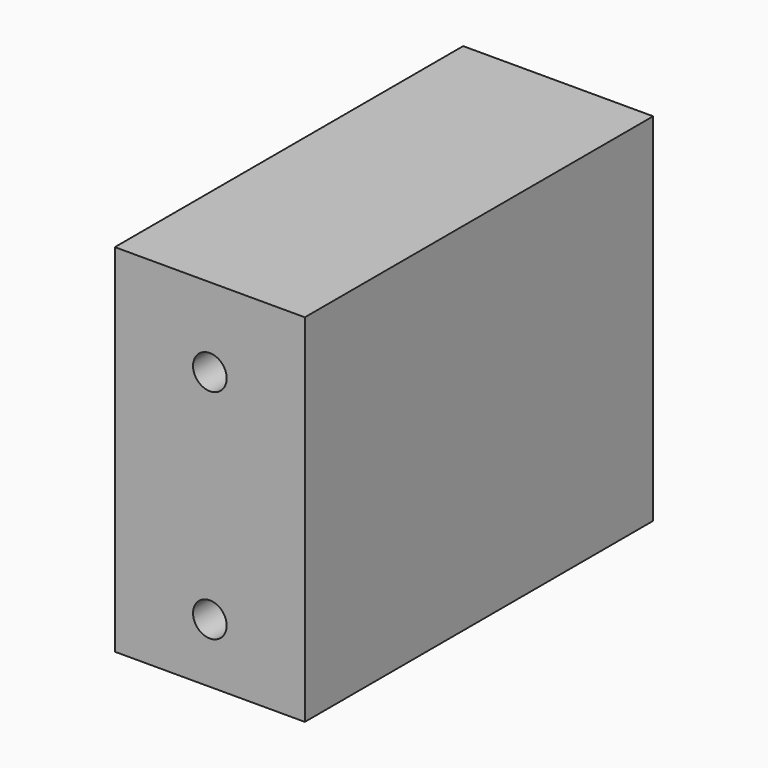
from build123d import *

# Parameters (mm, degrees)
F0_W     = 48
F0_H     = 90
F1_DEPTH = 110
F3_D     = 8.5


# Not quite as in the source:
# - the program builds the solid bodies; features that only make, move or delete a surface that nothing else refers to are left out


with BuildPart() as f1:
    # F0 (on Front) → F1 (new body)
    with BuildSketch(Plane.XZ):
        with Locations((24, 45)):
            Rectangle(F0_W, F0_H)
    extrude(amount=F1_DEPTH)

    # F3 (through all)
    with Locations(Plane.XZ.offset(110)):
        with Locations((24, 70), (24, 15)):
            Hole(F3_D / 2)


solid = f1.part
